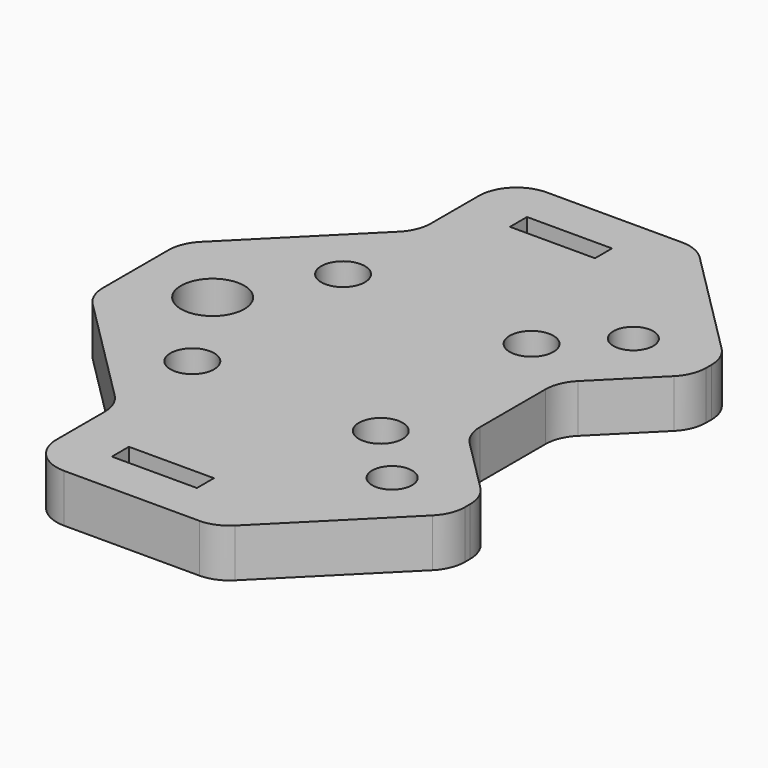
from build123d import *

# Parameters (mm, degrees)
F0_R     = 1.6
F0_W     = 11.2785340156
F0_H     = 2.8266120087
F0_R_2   = 2.65
F0_R_3   = 4.2
F1_DEPTH = 6.4
F2_R     = 5
F3_R     = 2.9
F4_DEPTH = 3.2


# Not quite as in the source:
# - a feature names something its author has since deleted; it is built from what else it names


with BuildPart() as f1:
    # F0 (on Top) → F1 (new body)
    with BuildSketch(Plane.XY):
        Polygon((-12.5, -40), (12.5, -40), (30, -22.5), (30, -17.5), (20, -7.5), (20, 7.5), (30, 17.5), (30, 22.5), (12.5, 40), (-12.5, 40), (-12.5, 25), (-30, 7.5), (-30, -7.5), (-12.5, -25), align=None)
        with Locations((-12.5, -12.5)):
            Circle(F0_R, mode=Mode.SUBTRACT)
        with Locations((0, -33)):
            Rectangle(F0_W, F0_H, mode=Mode.SUBTRACT)
        with Locations((12.5, -12.5)):
            Circle(F0_R, mode=Mode.SUBTRACT)
        with Locations((20, -20)):
            Circle(F0_R_2, mode=Mode.SUBTRACT)
        with Locations((-19.8, 0)):
            Circle(F0_R_3, mode=Mode.SUBTRACT)
        with Locations((-12.5, 12.5)):
            Circle(F0_R, mode=Mode.SUBTRACT)
        with Locations((12.5, 12.5)):
            Circle(F0_R, mode=Mode.SUBTRACT)
        with Locations((0, 33)):
            Rectangle(F0_W, F0_H, mode=Mode.SUBTRACT)
        with Locations((20, 20)):
            Circle(F0_R_2, mode=Mode.SUBTRACT)
    extrude(amount=F1_DEPTH)

    # F2
    f2_edges = [f1.edges().sort_by_distance(p)[0] for p in [
        (30, 17.5, 3.2),
        (30, 22.5, 3.2),
        (-12.5, -25, 3.2),
        (-12.5, 25, 3.2),
        (-12.5, -40, 3.2),
        (12.5, -40, 3.2),
        (30, -22.5, 3.2),
        (30, -17.5, 3.2),
        (20, -7.5, 3.2),
        (20, 7.5, 3.2),
        (12.5, 40, 3.2),
        (-12.5, 40, 3.2),
        (-30, 7.5, 3.2),
        (-30, -7.5, 3.2),
    ]]
    fillet(f2_edges, radius=F2_R)

    # F3 (on face) → F4 (cut)
    with BuildSketch(Plane.XY.offset(6.4)):
        with Locations((-12.5, 12.5)):
            Circle(F3_R)
        with Locations((12.5, 12.5)):
            Circle(F3_R)
        with Locations((12.5, -12.5)):
            Circle(F3_R)
        with Locations((-12.5, -12.5)):
            Circle(F3_R)
    extrude(amount=-F4_DEPTH, mode=Mode.SUBTRACT)


solid = f1.part
